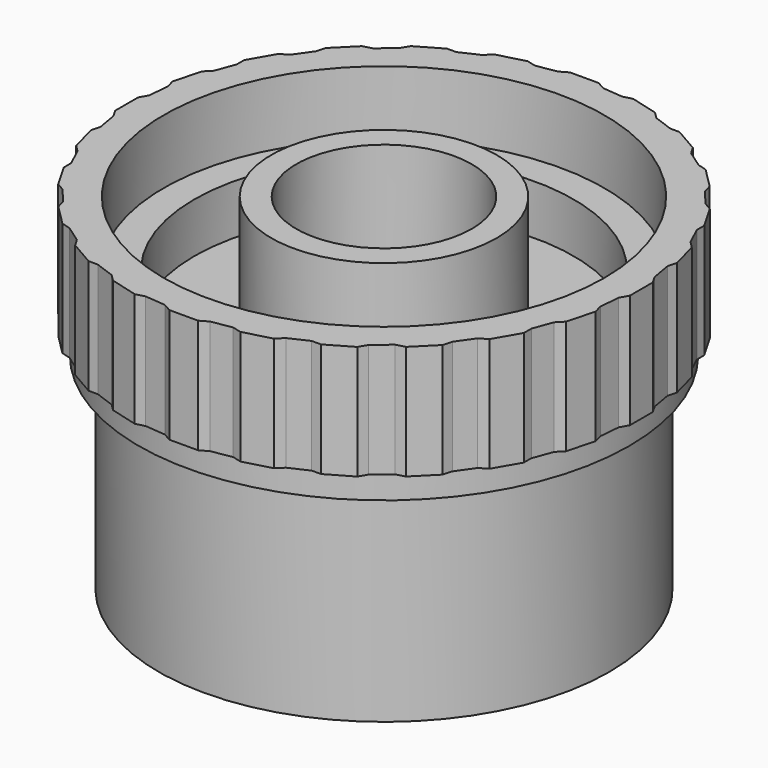
from build123d import *

# Parameters (mm, degrees)
F0_R      = 17.2
F0_R_2    = 15.45
F1_DEPTH  = 8
F0_R_3    = 13.3
F2_DEPTH  = 3.5
F0_R_4    = 7.9
F0_R_5    = 6.15
F3_DEPTH  = 8
F4_DEPTH  = 1.8
F5_R      = 15.8
F5_R_2    = 15.1
F6_DEPTH  = 14.4
F7_R      = 7.9
F7_R_2    = 6.15
F8_DEPTH  = 3
F9_DEPTH  = 25
F12_DEPTH = 8
F13_R     = 15.1
F14_DEPTH = 0.4
F15_DEPTH = 14


with BuildPart() as f1:
    # F0 (on Top) → F1 (new body)
    with BuildSketch(Plane.XY):
        Circle(F0_R)
        Circle(F0_R_2, mode=Mode.SUBTRACT)
    extrude(amount=F1_DEPTH)

    # F0 (on Top) → F2 (join)
    with BuildSketch(Plane.XY):
        Circle(F0_R_2)
        Circle(F0_R_3, mode=Mode.SUBTRACT)
    extrude(amount=F2_DEPTH)

    # F11 (on face) → F12 (join)
    with BuildSketch(Plane.XY.offset(8)):
        Polygon((-17.2313860185, 2.1472887428), (-16.613924199, 4.451687625), (-16.1184641245, 6.3007697959), (-16.5807553746, 5.8311789369), (-17.0430466247, 5.3615880779), (-17.5625070925, 3.4229352194), (-17.3969465555, 2.7851119811), align=None)
        Polygon((-17.2, 1.9143107781), (-17.2313860185, 2.1472887428), (-17.3969465555, 2.7851119811), (-17.525, 1.3410710597), align=None)
        with BuildLine():
            ThreePointArc((-17.2, 0), (-17.0528516123, 2.2450505314), (-16.613924199, 4.451687625))
            Line((-16.613924199, 4.451687625), (-17.2313860185, 2.1472887428))
            Line((-17.2313860185, 2.1472887428), (-17.2, 1.9143107781))
            Line((-17.2, 1.9143107781), (-17.2, 0))
        make_face()
        Polygon((-17.2, -2.3856892219), (-17.2, 0), (-17.2, 1.9143107781), (-17.525, 1.3410710597), (-17.85, 0.7678313414), (-17.85, -1.2392097851), (-17.525, -1.8124495035), align=None)
        Polygon((-17.1093842998, -2.6026053556), (-17.2, -2.3856892219), (-17.525, -1.8124495035), (-17.2749448368, -3.2404285939), align=None)
        Polygon((-15.9964624059, -6.7560864087), (-16.6139242133, -4.4516875717), (-17.1093842998, -2.6026053556), (-17.2749448368, -3.2404285939), (-17.4405053738, -3.8782518322), (-16.921044906, -5.8169046907), (-16.4587536559, -6.2864955497), align=None)
        with BuildLine():
            ThreePointArc((-16.6139242133, -4.4516875717), (-17.0528516159, -2.2450505041), (-17.2, 0))
            Line((-17.2, 0), (-17.2, -2.3856892219))
            Line((-17.2, -2.3856892219), (-17.1093842998, -2.6026053556))
            Line((-17.1093842998, -2.6026053556), (-16.6139242133, -4.4516875717))
        make_face()
        with BuildLine():
            ThreePointArc((-14.8956369049, -8.6000000696), (-15.8907279446, -6.5821550719), (-16.6139242133, -4.4516875717))
            Line((-16.6139242133, -4.4516875717), (-15.9964624059, -6.7560864087))
            Line((-15.9964624059, -6.7560864087), (-15.8527923342, -6.9421582354))
            Line((-15.8527923342, -6.9421582354), (-14.8956369049, -8.6000000696))
        make_face()
        Polygon((-15.8527923342, -6.9421582354), (-15.9964624059, -6.7560864087), (-16.4587536559, -6.2864955497), (-15.8476307312, -7.601098394), align=None)
        Polygon((-13.7027923342, -10.6660674717), (-14.8956369049, -8.6000000696), (-15.8527923342, -6.9421582354), (-15.8476307312, -7.601098394), (-15.8424691282, -8.2600385526), (-14.838948565, -9.9981871545), (-14.2708704496, -10.3321273131), align=None)
        with BuildLine():
            ThreePointArc((-12.1622366374, -12.1622366354), (-13.6456774289, -10.4706966103), (-14.8956369049, -8.6000000696))
            Line((-14.8956369049, -8.6000000696), (-13.7027923342, -10.6660674717))
            Line((-13.7027923342, -10.6660674717), (-13.5158587689, -10.8086145039))
            Line((-13.5158587689, -10.8086145039), (-12.1622366374, -12.1622366354))
        make_face()
        Polygon((-13.5158587689, -10.8086145039), (-13.7027923342, -10.6660674717), (-14.2708704496, -10.3321273131), (-13.3403267807, -11.4437658999), align=None)
        Polygon((-10.4752996098, -13.849173663), (-12.1622366374, -12.1622366354), (-13.5158587689, -10.8086145039), (-13.3403267807, -11.4437658999), (-13.1647947925, -12.0789172959), (-11.7456024018, -13.4981096866), (-11.1104510058, -13.6736416748), align=None)
        with BuildLine():
            ThreePointArc((-8.5999995119, -14.8956372269), (-10.4706963559, -13.6456776241), (-12.1622366374, -12.1622366354))
            Line((-12.1622366374, -12.1622366354), (-10.4752996098, -13.849173663))
            Line((-10.4752996098, -13.849173663), (-10.2578417646, -13.938481556))
            Line((-10.2578417646, -13.938481556), (-8.5999995119, -14.8956372269))
        make_face()
        Polygon((-10.2578417646, -13.938481556), (-10.4752996098, -13.849173663), (-11.1104510058, -13.6736416748), (-9.923901606, -14.5065596715), align=None)
        Polygon((-6.5339325283, -16.088481556), (-8.5999995119, -14.8956372269), (-10.2578417646, -13.938481556), (-9.923901606, -14.5065596715), (-9.5899614474, -15.0746377869), (-7.8518128455, -16.0781583501), (-7.1928726869, -16.0833199531), align=None)
        Polygon((-2.1472887428, -17.2313860185), (-4.451687625, -16.613924199), (-6.3007697959, -16.1184641245), (-5.8311789369, -16.5807553746), (-5.3615880779, -17.0430466247), (-3.4229352194, -17.5625070925), (-2.7851119811, -17.3969465555), align=None)
        Polygon((-6.3007697959, -16.1184641245), (-6.5339325283, -16.088481556), (-7.1928726869, -16.0833199531), (-5.8311789369, -16.5807553746), align=None)
        with BuildLine():
            ThreePointArc((-4.451687625, -16.613924199), (-6.5821547999, -15.8907280573), (-8.5999995119, -14.8956372269))
            Line((-8.5999995119, -14.8956372269), (-6.5339325283, -16.088481556))
            Line((-6.5339325283, -16.088481556), (-6.3007697959, -16.1184641245))
            Line((-6.3007697959, -16.1184641245), (-4.451687625, -16.613924199))
        make_face()
        with BuildLine():
            ThreePointArc((0, -17.2), (-2.2450505314, -17.0528516123), (-4.451687625, -16.613924199))
            Line((-4.451687625, -16.613924199), (-2.1472887428, -17.2313860185))
            Line((-2.1472887428, -17.2313860185), (-1.9143107781, -17.2))
            Line((-1.9143107781, -17.2), (0, -17.2))
        make_face()
        Polygon((2.3856892219, -17.2), (0, -17.2), (-1.9143107781, -17.2), (-1.3410710597, -17.525), (-0.7678313414, -17.85), (1.2392097851, -17.85), (1.8124495035, -17.525), align=None)
        Polygon((-1.9143107781, -17.2), (-2.1472887428, -17.2313860185), (-2.7851119811, -17.3969465555), (-1.3410710597, -17.525), align=None)
        with BuildLine():
            Line((2.6026053556, -17.1093842998), (4.4516877488, -16.6139241658))
            ThreePointArc((4.4516877488, -16.6139241658), (2.245050595, -17.0528516039), (0, -17.2))
            Line((0, -17.2), (2.3856892219, -17.2))
            Line((2.3856892219, -17.2), (2.6026053556, -17.1093842998))
        make_face()
        Polygon((3.2404285939, -17.2749448368), (2.6026053556, -17.1093842998), (2.3856892219, -17.2), (1.8124495035, -17.525), align=None)
        Polygon((6.7560864087, -15.9964624059), (4.4516877488, -16.6139241658), (2.6026053556, -17.1093842998), (3.2404285939, -17.2749448368), (3.8782518322, -17.4405053738), (5.8169046907, -16.921044906), (6.2864955497, -16.4587536559), align=None)
        with BuildLine():
            Line((6.9421582354, -15.8527923342), (8.6000001368, -14.8956368661))
            ThreePointArc((8.6000001368, -14.8956368661), (6.5821551924, -15.8907278947), (4.4516877488, -16.6139241658))
            Line((4.4516877488, -16.6139241658), (6.7560864087, -15.9964624059))
            Line((6.7560864087, -15.9964624059), (6.9421582354, -15.8527923342))
        make_face()
        Polygon((7.601098394, -15.8476307312), (6.9421582354, -15.8527923342), (6.7560864087, -15.9964624059), (6.2864955497, -16.4587536559), align=None)
        Polygon((10.6660674717, -13.7027923342), (8.6000001368, -14.8956368661), (6.9421582354, -15.8527923342), (7.601098394, -15.8476307312), (8.2600385526, -15.8424691282), (9.9981871545, -14.838948565), (10.3321273131, -14.2708704496), align=None)
        Polygon((13.849173663, -10.4752996098), (12.1622366354, -12.1622366374), (10.8086145039, -13.5158587689), (11.4437658999, -13.3403267807), (12.0789172959, -13.1647947925), (13.4981096866, -11.7456024018), (13.6736416748, -11.1104510058), align=None)
        Polygon((11.4437658999, -13.3403267807), (10.8086145039, -13.5158587689), (10.6660674717, -13.7027923342), (10.3321273131, -14.2708704496), align=None)
        with BuildLine():
            Line((10.8086145039, -13.5158587689), (12.1622366354, -12.1622366374))
            ThreePointArc((12.1622366354, -12.1622366374), (10.470696641, -13.6456774054), (8.6000001368, -14.8956368661))
            Line((8.6000001368, -14.8956368661), (10.6660674717, -13.7027923342))
            Line((10.6660674717, -13.7027923342), (10.8086145039, -13.5158587689))
        make_face()
        with BuildLine():
            Line((13.938481556, -10.2578417646), (14.8956372269, -8.5999995119))
            ThreePointArc((14.8956372269, -8.5999995119), (13.6456776241, -10.4706963559), (12.1622366354, -12.1622366374))
            Line((12.1622366354, -12.1622366374), (13.849173663, -10.4752996098))
            Line((13.849173663, -10.4752996098), (13.938481556, -10.2578417646))
        make_face()
        Polygon((14.5065596715, -9.923901606), (13.938481556, -10.2578417646), (13.849173663, -10.4752996098), (13.6736416748, -11.1104510058), align=None)
        Polygon((16.088481556, -6.5339325283), (14.8956372269, -8.5999995119), (13.938481556, -10.2578417646), (14.5065596715, -9.923901606), (15.0746377869, -9.5899614474), (16.0781583501, -7.8518128455), (16.0833199531, -7.1928726869), align=None)
        with BuildLine():
            Line((16.1184641245, -6.3007697959), (16.6139242465, -4.4516874478))
            ThreePointArc((16.6139242465, -4.4516874478), (15.8907280924, -6.5821547151), (14.8956372269, -8.5999995119))
            Line((14.8956372269, -8.5999995119), (16.088481556, -6.5339325283))
            Line((16.088481556, -6.5339325283), (16.1184641245, -6.3007697959))
        make_face()
        Polygon((16.5807553746, -5.8311789369), (16.1184641245, -6.3007697959), (16.088481556, -6.5339325283), (16.0833199531, -7.1928726869), align=None)
        Polygon((17.2313860185, -2.1472887428), (16.6139242465, -4.4516874478), (16.1184641245, -6.3007697959), (16.5807553746, -5.8311789369), (17.0430466247, -5.3615880779), (17.5625070925, -3.4229352194), (17.3969465555, -2.7851119811), align=None)
        with BuildLine():
            Line((17.2, -1.9143107781), (17.2, 0))
            ThreePointArc((17.2, 0), (17.0528516243, -2.2450504405), (16.6139242465, -4.4516874478))
            Line((16.6139242465, -4.4516874478), (17.2313860185, -2.1472887428))
            Line((17.2313860185, -2.1472887428), (17.2, -1.9143107781))
        make_face()
        Polygon((17.525, -1.3410710597), (17.2, -1.9143107781), (17.2313860185, -2.1472887428), (17.3969465555, -2.7851119811), align=None)
        Polygon((17.2, 2.3856892219), (17.2, 0), (17.2, -1.9143107781), (17.525, -1.3410710597), (17.85, -0.7678313414), (17.85, 1.2392097851), (17.525, 1.8124495035), align=None)
        with BuildLine():
            Line((17.1093842998, 2.6026053556), (16.61392429, 4.4516872853))
            ThreePointArc((16.61392429, 4.4516872853), (17.0528516353, 2.2450503571), (17.2, 0))
            Line((17.2, 0), (17.2, 2.3856892219))
            Line((17.2, 2.3856892219), (17.1093842998, 2.6026053556))
        make_face()
        Polygon((17.2749448368, 3.2404285939), (17.1093842998, 2.6026053556), (17.2, 2.3856892219), (17.525, 1.8124495035), align=None)
        Polygon((15.9964624059, 6.7560864087), (16.61392429, 4.4516872853), (17.1093842998, 2.6026053556), (17.2749448368, 3.2404285939), (17.4405053738, 3.8782518322), (16.921044906, 5.8169046907), (16.4587536559, 6.2864955497), align=None)
        with BuildLine():
            Line((15.8527923342, 6.9421582354), (14.8956368594, 8.6000001484))
            ThreePointArc((14.8956368594, 8.6000001484), (15.8907279839, 6.5821549769), (16.61392429, 4.4516872853))
            Line((16.61392429, 4.4516872853), (15.9964624059, 6.7560864087))
            Line((15.9964624059, 6.7560864087), (15.8527923342, 6.9421582354))
        make_face()
        Polygon((15.8476307312, 7.601098394), (15.8527923342, 6.9421582354), (15.9964624059, 6.7560864087), (16.4587536559, 6.2864955497), align=None)
        Polygon((13.7027923342, 10.6660674717), (14.8956368594, 8.6000001484), (15.8527923342, 6.9421582354), (15.8476307312, 7.601098394), (15.8424691282, 8.2600385526), (14.838948565, 9.9981871545), (14.2708704496, 10.3321273131), align=None)
        with BuildLine():
            Line((13.5158587689, 10.8086145039), (12.1622365879, 12.1622366849))
            ThreePointArc((12.1622365879, 12.1622366849), (13.6456773799, 10.4706966742), (14.8956368594, 8.6000001484))
            Line((14.8956368594, 8.6000001484), (13.7027923342, 10.6660674717))
            Line((13.7027923342, 10.6660674717), (13.5158587689, 10.8086145039))
        make_face()
        Polygon((13.3403267807, 11.4437658999), (13.5158587689, 10.8086145039), (13.7027923342, 10.6660674717), (14.2708704496, 10.3321273131), align=None)
        Polygon((10.4752996098, 13.849173663), (12.1622365879, 12.1622366849), (13.5158587689, 10.8086145039), (13.3403267807, 11.4437658999), (13.1647947925, 12.0789172959), (11.7456024018, 13.4981096866), (11.1104510058, 13.6736416748), align=None)
        with BuildLine():
            Line((10.2578417646, 13.938481556), (8.5999994254, 14.8956372768))
            ThreePointArc((8.5999994254, 14.8956372768), (10.4706962885, 13.6456776759), (12.1622365879, 12.1622366849))
            Line((12.1622365879, 12.1622366849), (10.4752996098, 13.849173663))
            Line((10.4752996098, 13.849173663), (10.2578417646, 13.938481556))
        make_face()
        Polygon((9.923901606, 14.5065596715), (10.2578417646, 13.938481556), (10.4752996098, 13.849173663), (11.1104510058, 13.6736416748), align=None)
        Polygon((6.5339325283, 16.088481556), (8.5999994254, 14.8956372768), (10.2578417646, 13.938481556), (9.923901606, 14.5065596715), (9.5899614474, 15.0746377869), (7.8518128455, 16.0781583501), (7.1928726869, 16.0833199531), align=None)
        with BuildLine():
            Line((6.3007697959, 16.1184641245), (4.4516875681, 16.6139242142))
            ThreePointArc((4.4516875681, 16.6139242142), (6.5821547265, 15.8907280877), (8.5999994254, 14.8956372768))
            Line((8.5999994254, 14.8956372768), (6.5339325283, 16.088481556))
            Line((6.5339325283, 16.088481556), (6.3007697959, 16.1184641245))
        make_face()
        Polygon((5.8311789369, 16.5807553746), (6.3007697959, 16.1184641245), (6.5339325283, 16.088481556), (7.1928726869, 16.0833199531), align=None)
        Polygon((2.1472887428, 17.2313860185), (4.4516875681, 16.6139242142), (6.3007697959, 16.1184641245), (5.8311789369, 16.5807553746), (5.3615880779, 17.0430466247), (3.4229352194, 17.5625070925), (2.7851119811, 17.3969465555), align=None)
        with BuildLine():
            Line((1.9143107781, 17.2), (0, 17.2))
            ThreePointArc((0, 17.2), (2.2450505022, 17.0528516161), (4.4516875681, 16.6139242142))
            Line((4.4516875681, 16.6139242142), (2.1472887428, 17.2313860185))
            Line((2.1472887428, 17.2313860185), (1.9143107781, 17.2))
        make_face()
        Polygon((1.3410710597, 17.525), (1.9143107781, 17.2), (2.1472887428, 17.2313860185), (2.7851119811, 17.3969465555), align=None)
        Polygon((-1.8124495035, 17.525), (-2.3856892219, 17.2), (0, 17.2), (1.9143107781, 17.2), (1.3410710597, 17.525), (0.7678313414, 17.85), (-1.2392097851, 17.85), align=None)
        with BuildLine():
            Line((0, 17.2), (-2.3856892219, 17.2))
            Line((-2.3856892219, 17.2), (-2.6026053556, 17.1093842998))
            Line((-2.6026053556, 17.1093842998), (-4.4516875299, 16.6139242244))
            ThreePointArc((-4.4516875299, 16.6139242244), (-2.2450504827, 17.0528516187), (0, 17.2))
        make_face()
        Polygon((-2.6026053556, 17.1093842998), (-2.3856892219, 17.2), (-1.8124495035, 17.525), (-3.2404285939, 17.2749448368), align=None)
        Polygon((-4.4516875299, 16.6139242244), (-2.6026053556, 17.1093842998), (-3.2404285939, 17.2749448368), (-3.8782518322, 17.4405053738), (-5.8169046907, 16.921044906), (-6.2864955497, 16.4587536559), (-6.7560864087, 15.9964624059), align=None)
        with BuildLine():
            ThreePointArc((-8.6000001201, 14.8956368757), (-6.5821550788, 15.8907279417), (-4.4516875299, 16.6139242244))
            Line((-4.4516875299, 16.6139242244), (-6.7560864087, 15.9964624059))
            Line((-6.7560864087, 15.9964624059), (-6.9421582354, 15.8527923342))
            Line((-6.9421582354, 15.8527923342), (-8.6000001201, 14.8956368757))
        make_face()
        Polygon((-6.9421582354, 15.8527923342), (-6.7560864087, 15.9964624059), (-6.2864955497, 16.4587536559), (-7.601098394, 15.8476307312), align=None)
        Polygon((-10.6660674717, 13.7027923342), (-8.6000001201, 14.8956368757), (-6.9421582354, 15.8527923342), (-7.601098394, 15.8476307312), (-8.2600385526, 15.8424691282), (-9.9981871545, 14.838948565), (-10.3321273131, 14.2708704496), align=None)
        with BuildLine():
            ThreePointArc((-12.1622366354, 12.1622366374), (-10.4706966334, 13.6456774112), (-8.6000001201, 14.8956368757))
            Line((-8.6000001201, 14.8956368757), (-10.6660674717, 13.7027923342))
            Line((-10.6660674717, 13.7027923342), (-10.8086145039, 13.5158587689))
            Line((-10.8086145039, 13.5158587689), (-12.1622366354, 12.1622366374))
        make_face()
        Polygon((-10.8086145039, 13.5158587689), (-10.6660674717, 13.7027923342), (-10.3321273131, 14.2708704496), (-11.4437658999, 13.3403267807), align=None)
        Polygon((-13.849173663, 10.4752996098), (-12.1622366354, 12.1622366374), (-10.8086145039, 13.5158587689), (-11.4437658999, 13.3403267807), (-12.0789172959, 13.1647947925), (-13.4981096866, 11.7456024018), (-13.6736416748, 11.1104510058), align=None)
        with BuildLine():
            ThreePointArc((-14.895637301, 8.5999993835), (-13.6456776693, 10.4706962971), (-12.1622366354, 12.1622366374))
            Line((-12.1622366354, 12.1622366374), (-13.849173663, 10.4752996098))
            Line((-13.849173663, 10.4752996098), (-13.938481556, 10.2578417646))
            Line((-13.938481556, 10.2578417646), (-14.895637301, 8.5999993835))
        make_face()
        Polygon((-13.938481556, 10.2578417646), (-13.849173663, 10.4752996098), (-13.6736416748, 11.1104510058), (-14.5065596715, 9.923901606), align=None)
        Polygon((-16.088481556, 6.5339325283), (-14.895637301, 8.5999993835), (-13.938481556, 10.2578417646), (-14.5065596715, 9.923901606), (-15.0746377869, 9.5899614474), (-16.0781583501, 7.8518128455), (-16.0833199531, 7.1928726869), align=None)
        with BuildLine():
            ThreePointArc((-16.613924199, 4.451687625), (-15.8907280857, 6.5821547314), (-14.895637301, 8.5999993835))
            Line((-14.895637301, 8.5999993835), (-16.088481556, 6.5339325283))
            Line((-16.088481556, 6.5339325283), (-16.1184641245, 6.3007697959))
            Line((-16.1184641245, 6.3007697959), (-16.613924199, 4.451687625))
        make_face()
        Polygon((-16.1184641245, 6.3007697959), (-16.088481556, 6.5339325283), (-16.0833199531, 7.1928726869), (-16.5807553746, 5.8311789369), align=None)
    extrude(amount=-F12_DEPTH)


with BuildPart() as f3:
    # F0 (on Top) → F3 (new body)
    with BuildSketch(Plane.XY):
        Circle(F0_R_4)
        Circle(F0_R_5, mode=Mode.SUBTRACT)
    extrude(amount=F3_DEPTH)


with BuildPart() as f4:
    # F0 (on Top) → F4 (new body)
    with BuildSketch(Plane.XY):
        Circle(F0_R)
        Circle(F0_R_2, mode=Mode.SUBTRACT)
        Circle(F0_R_2)
        Circle(F0_R_3, mode=Mode.SUBTRACT)
        Circle(F0_R_3)
        Circle(F0_R_4, mode=Mode.SUBTRACT)
        Circle(F0_R_4)
        Circle(F0_R_5, mode=Mode.SUBTRACT)
        Circle(F0_R_5)
    extrude(amount=-F4_DEPTH)

    # F5 (on face) → F6 (join)
    with BuildSketch(Plane(origin=(0, 0, -1.8), x_dir=(1, 0, 0), z_dir=(0, 0, -1))):
        Circle(F5_R)
        Circle(F5_R_2, mode=Mode.SUBTRACT)
    extrude(amount=F6_DEPTH)

    # F7 (on face) → F8 (join)
    with BuildSketch(Plane(origin=(0, 0, -1.8), x_dir=(1, 0, 0), z_dir=(0, 0, -1))):
        Circle(F7_R)
        Circle(F7_R_2, mode=Mode.SUBTRACT)
    extrude(amount=F8_DEPTH)

    # F9 (cut): a face of the model
    f9_faces = [f4.faces().sort_by_distance(p)[0] for p in [
        (0, 0, -1.8),
    ]]
    extrude(f9_faces, amount=-F9_DEPTH, mode=Mode.SUBTRACT)


with BuildPart() as f14:
    # F13 (on face) → F14 (new body)
    with BuildSketch(Plane(origin=(0, 0, -16.2), x_dir=(1, 0, 0), z_dir=(0, 0, -1))):
        Circle(F13_R)
        with BuildLine():
            Line((-1.3541611635, 13.3700582353), (-0.2968639122, 11.6420455351))
            Line((-0.2968639122, 11.6420455351), (0.6709903586, 13.4216981642))
            ThreePointArc((0.6709903586, 13.4216981642), (0.8730116488, 13.6229593891), (1.1521957346, 13.681053525))
            ThreePointArc((1.1521957346, 13.681053525), (1.4444908929, 13.653286294), (1.736125432, 13.6192749091))
            ThreePointArc((1.736125432, 13.6192749091), (1.9969723384, 13.5040465541), (2.1524064647, 13.2649672477))
            Line((2.1524064647, 13.2649672477), (2.7264345888, 11.3221864874))
            Line((2.7264345888, 11.3221864874), (4.1219180191, 12.7906998055))
            ThreePointArc((4.1219180191, 12.7906998055), (4.3691458388, 12.9328162631), (4.6538528263, 12.9166727308))
            ThreePointArc((4.6538528263, 12.9166727308), (4.9290015804, 12.8142000915), (5.2018961194, 12.7058670435))
            ThreePointArc((5.2018961194, 12.7058670435), (5.4240315902, 12.5270528523), (5.5122911492, 12.2558906636))
            Line((5.5122911492, 12.2558906636), (5.5639310781, 10.2307391415))
            Line((5.5639310781, 10.2307391415), (7.2919437783, 11.2880363928))
            ThreePointArc((7.2919437783, 11.2880363928), (7.5675299602, 11.3613230813), (7.8383575388, 11.2720420359))
            ThreePointArc((7.8383575388, 11.2720420359), (8.0776089558, 11.1018473293), (8.3131661828, 10.9265753364))
            ThreePointArc((8.3131661828, 10.9265753364), (8.4814520528, 10.6963612005), (8.4965223015, 10.4115953845))
            Line((8.4965223015, 10.4115953845), (8.0222548594, 8.4420838301))
            Line((8.0222548594, 8.4420838301), (9.9650356196, 9.0161119542))
            ThreePointArc((9.9650356196, 9.0161119542), (10.2501994208, 9.0155745069), (10.4886911385, 8.8592403041))
            ThreePointArc((10.4886911385, 8.8592403041), (10.6757406297, 8.6329220182), (10.857907709, 8.4026555771))
            ThreePointArc((10.857907709, 8.4026555771), (10.9608755742, 8.1367302095), (10.9017295001, 7.857767086))
            Line((10.9017295001, 7.857767086), (9.9338752293, 6.0781144569))
            Line((9.9338752293, 6.0781144569), (11.9590267514, 6.1297543858))
            ThreePointArc((11.9590267514, 6.1297543858), (12.2343347301, 6.0554294289), (12.4242377705, 5.8426959862))
            ThreePointArc((12.4242377705, 5.8426959862), (12.5463382222, 5.5756773382), (12.6627007684, 5.3061087262))
            ThreePointArc((12.6627007684, 5.3061087262), (12.693333539, 5.0225945013), (12.5640018492, 4.7684449462))
            Line((12.5640018492, 4.7684449462), (11.1685184189, 3.2999316281))
            Line((11.1685184189, 3.2999316281), (13.1380299733, 2.8256641859))
            ThreePointArc((13.1380299733, 2.8256641859), (13.3847203457, 2.6826168423), (13.5130931304, 2.4279815924))
            ThreePointArc((13.5130931304, 2.4279815924), (13.5619235986, 2.1384594618), (13.6045516965, 1.8479593345))
            ThreePointArc((13.6045516965, 1.8479593345), (13.5607617998, 1.5661772781), (13.3700582353, 1.3541611635))
            Line((13.3700582353, 1.3541611635), (11.6420455351, 0.2968639122))
            Line((11.6420455351, 0.2968639122), (13.4216981642, -0.6709903586))
            ThreePointArc((13.4216981642, -0.6709903586), (13.6229593891, -0.8730116488), (13.681053525, -1.1521957346))
            ThreePointArc((13.681053525, -1.1521957346), (13.653286294, -1.4444908929), (13.6192749091, -1.736125432))
            ThreePointArc((13.6192749091, -1.736125432), (13.5040465541, -1.9969723384), (13.2649672477, -2.1524064647))
            Line((13.2649672477, -2.1524064647), (11.3221864874, -2.7264345888))
            Line((11.3221864874, -2.7264345888), (12.7906998055, -4.1219180191))
            ThreePointArc((12.7906998055, -4.1219180191), (12.9328162631, -4.3691458388), (12.9166727308, -4.6538528263))
            ThreePointArc((12.9166727308, -4.6538528263), (12.8142000915, -4.9290015804), (12.7058670435, -5.2018961194))
            ThreePointArc((12.7058670435, -5.2018961194), (12.5270528523, -5.4240315902), (12.2558906636, -5.5122911492))
            Line((12.2558906636, -5.5122911492), (10.2307391415, -5.5639310781))
            Line((10.2307391415, -5.5639310781), (11.2880363928, -7.2919437783))
            ThreePointArc((11.2880363928, -7.2919437783), (11.3613230813, -7.5675299602), (11.2720420359, -7.8383575388))
            ThreePointArc((11.2720420359, -7.8383575388), (11.1018473293, -8.0776089558), (10.9265753364, -8.3131661828))
            ThreePointArc((10.9265753364, -8.3131661828), (10.6963612005, -8.4814520528), (10.4115953845, -8.4965223015))
            Line((10.4115953845, -8.4965223015), (8.4420838301, -8.0222548594))
            Line((8.4420838301, -8.0222548594), (9.0161119542, -9.9650356196))
            ThreePointArc((9.0161119542, -9.9650356196), (9.0155745069, -10.2501994208), (8.8592403041, -10.4886911385))
            ThreePointArc((8.8592403041, -10.4886911385), (8.6329220182, -10.6757406297), (8.4026555771, -10.857907709))
            ThreePointArc((8.4026555771, -10.857907709), (8.1367302095, -10.9608755742), (7.857767086, -10.9017295001))
            Line((7.857767086, -10.9017295001), (6.0781144569, -9.9338752293))
            Line((6.0781144569, -9.9338752293), (6.1297543858, -11.9590267514))
            ThreePointArc((6.1297543858, -11.9590267514), (6.0554294289, -12.2343347301), (5.8426959862, -12.4242377705))
            ThreePointArc((5.8426959862, -12.4242377705), (5.5756773382, -12.5463382222), (5.3061087262, -12.6627007684))
            ThreePointArc((5.3061087262, -12.6627007684), (5.0225945013, -12.693333539), (4.7684449462, -12.5640018492))
            Line((4.7684449462, -12.5640018492), (3.2999316281, -11.1685184189))
            Line((3.2999316281, -11.1685184189), (2.8256641859, -13.1380299733))
            ThreePointArc((2.8256641859, -13.1380299733), (2.6826168423, -13.3847203457), (2.4279815924, -13.5130931304))
            ThreePointArc((2.4279815924, -13.5130931304), (2.1384594618, -13.5619235986), (1.8479593345, -13.6045516965))
            ThreePointArc((1.8479593345, -13.6045516965), (1.5661772781, -13.5607617998), (1.3541611635, -13.3700582353))
            Line((1.3541611635, -13.3700582353), (0.2968639122, -11.6420455351))
            Line((0.2968639122, -11.6420455351), (-0.6709903586, -13.4216981642))
            ThreePointArc((-0.6709903586, -13.4216981642), (-0.8730116488, -13.6229593891), (-1.1521957346, -13.681053525))
            ThreePointArc((-1.1521957346, -13.681053525), (-1.4444908929, -13.653286294), (-1.736125432, -13.6192749091))
            ThreePointArc((-1.736125432, -13.6192749091), (-1.9969723384, -13.5040465541), (-2.1524064647, -13.2649672477))
            Line((-2.1524064647, -13.2649672477), (-2.7264345888, -11.3221864874))
            Line((-2.7264345888, -11.3221864874), (-4.1219180191, -12.7906998055))
            ThreePointArc((-4.1219180191, -12.7906998055), (-4.3691458388, -12.9328162631), (-4.6538528263, -12.9166727308))
            ThreePointArc((-4.6538528263, -12.9166727308), (-4.9290015804, -12.8142000915), (-5.2018961194, -12.7058670435))
            ThreePointArc((-5.2018961194, -12.7058670435), (-5.4240315902, -12.5270528523), (-5.5122911492, -12.2558906636))
            Line((-5.5122911492, -12.2558906636), (-5.5639310781, -10.2307391415))
            Line((-5.5639310781, -10.2307391415), (-7.2919437783, -11.2880363928))
            ThreePointArc((-7.2919437783, -11.2880363928), (-7.5675299602, -11.3613230813), (-7.8383575388, -11.2720420359))
            ThreePointArc((-7.8383575388, -11.2720420359), (-8.0776089558, -11.1018473293), (-8.3131661828, -10.9265753364))
            ThreePointArc((-8.3131661828, -10.9265753364), (-8.4814520528, -10.6963612005), (-8.4965223015, -10.4115953845))
            Line((-8.4965223015, -10.4115953845), (-8.0222548594, -8.4420838301))
            Line((-8.0222548594, -8.4420838301), (-9.9650356196, -9.0161119542))
            ThreePointArc((-9.9650356196, -9.0161119542), (-10.2501994208, -9.0155745069), (-10.4886911385, -8.8592403041))
            ThreePointArc((-10.4886911385, -8.8592403041), (-10.6757406297, -8.6329220182), (-10.857907709, -8.4026555771))
            ThreePointArc((-10.857907709, -8.4026555771), (-10.9608755742, -8.1367302095), (-10.9017295001, -7.857767086))
            Line((-10.9017295001, -7.857767086), (-9.9338752293, -6.0781144569))
            Line((-9.9338752293, -6.0781144569), (-11.9590267514, -6.1297543858))
            ThreePointArc((-11.9590267514, -6.1297543858), (-12.2343347301, -6.0554294289), (-12.4242377705, -5.8426959862))
            ThreePointArc((-12.4242377705, -5.8426959862), (-12.5463382222, -5.5756773382), (-12.6627007684, -5.3061087262))
            ThreePointArc((-12.6627007684, -5.3061087262), (-12.693333539, -5.0225945013), (-12.5640018492, -4.7684449462))
            Line((-12.5640018492, -4.7684449462), (-11.1685184189, -3.2999316281))
            Line((-11.1685184189, -3.2999316281), (-13.1380299733, -2.8256641859))
            ThreePointArc((-13.1380299733, -2.8256641859), (-13.3847203457, -2.6826168423), (-13.5130931304, -2.4279815924))
            ThreePointArc((-13.5130931304, -2.4279815924), (-13.5619235986, -2.1384594618), (-13.6045516965, -1.8479593345))
            ThreePointArc((-13.6045516965, -1.8479593345), (-13.5607617998, -1.5661772781), (-13.3700582353, -1.3541611635))
            Line((-13.3700582353, -1.3541611635), (-11.6420455351, -0.2968639122))
            Line((-11.6420455351, -0.2968639122), (-13.4216981642, 0.6709903586))
            ThreePointArc((-13.4216981642, 0.6709903586), (-13.6229593891, 0.8730116488), (-13.681053525, 1.1521957346))
            ThreePointArc((-13.681053525, 1.1521957346), (-13.653286294, 1.4444908929), (-13.6192749091, 1.736125432))
            ThreePointArc((-13.6192749091, 1.736125432), (-13.5040465541, 1.9969723384), (-13.2649672477, 2.1524064647))
            Line((-13.2649672477, 2.1524064647), (-11.3221864874, 2.7264345888))
            Line((-11.3221864874, 2.7264345888), (-12.7906998055, 4.1219180191))
            ThreePointArc((-12.7906998055, 4.1219180191), (-12.9328162631, 4.3691458388), (-12.9166727308, 4.6538528263))
            ThreePointArc((-12.9166727308, 4.6538528263), (-12.8142000915, 4.9290015804), (-12.7058670435, 5.2018961194))
            ThreePointArc((-12.7058670435, 5.2018961194), (-12.5270528523, 5.4240315902), (-12.2558906636, 5.5122911492))
            Line((-12.2558906636, 5.5122911492), (-10.2307391415, 5.5639310781))
            Line((-10.2307391415, 5.5639310781), (-11.2880363928, 7.2919437783))
            ThreePointArc((-11.2880363928, 7.2919437783), (-11.3613230813, 7.5675299602), (-11.2720420359, 7.8383575388))
            ThreePointArc((-11.2720420359, 7.8383575388), (-11.1018473293, 8.0776089558), (-10.9265753364, 8.3131661828))
            ThreePointArc((-10.9265753364, 8.3131661828), (-10.6963612005, 8.4814520528), (-10.4115953845, 8.4965223015))
            Line((-10.4115953845, 8.4965223015), (-8.4420838301, 8.0222548594))
            Line((-8.4420838301, 8.0222548594), (-9.0161119542, 9.9650356196))
            ThreePointArc((-9.0161119542, 9.9650356196), (-9.0155745069, 10.2501994208), (-8.8592403041, 10.4886911385))
            ThreePointArc((-8.8592403041, 10.4886911385), (-8.6329220182, 10.6757406297), (-8.4026555771, 10.857907709))
            ThreePointArc((-8.4026555771, 10.857907709), (-8.1367302095, 10.9608755742), (-7.857767086, 10.9017295001))
            Line((-7.857767086, 10.9017295001), (-6.0781144569, 9.9338752293))
            Line((-6.0781144569, 9.9338752293), (-6.1297543858, 11.9590267514))
            ThreePointArc((-6.1297543858, 11.9590267514), (-6.0554294289, 12.2343347301), (-5.8426959862, 12.4242377705))
            ThreePointArc((-5.8426959862, 12.4242377705), (-5.5756773382, 12.5463382222), (-5.3061087262, 12.6627007684))
            ThreePointArc((-5.3061087262, 12.6627007684), (-5.0225945013, 12.693333539), (-4.7684449462, 12.5640018492))
            Line((-4.7684449462, 12.5640018492), (-3.2999316281, 11.1685184189))
            Line((-3.2999316281, 11.1685184189), (-2.8256641859, 13.1380299733))
            ThreePointArc((-2.8256641859, 13.1380299733), (-2.6826168423, 13.3847203457), (-2.4279815924, 13.5130931304))
            ThreePointArc((-2.4279815924, 13.5130931304), (-2.1384594618, 13.5619235986), (-1.8479593345, 13.6045516965))
            ThreePointArc((-1.8479593345, 13.6045516965), (-1.5661772781, 13.5607617998), (-1.3541611635, 13.3700582353))
        make_face(mode=Mode.SUBTRACT)
    extrude(amount=-F14_DEPTH)


with BuildPart() as f15:
    # F15 (new, through all): a face of the model
    f15_faces = [f14.part.faces().sort_by_distance(p)[0] for p in [
        (-14.6729075042, 0, -15.8),
    ]]
    extrude(f15_faces, amount=F15_DEPTH)


solid = Compound([f1.part, f3.part, f4.part, f14.part, f15.part])
